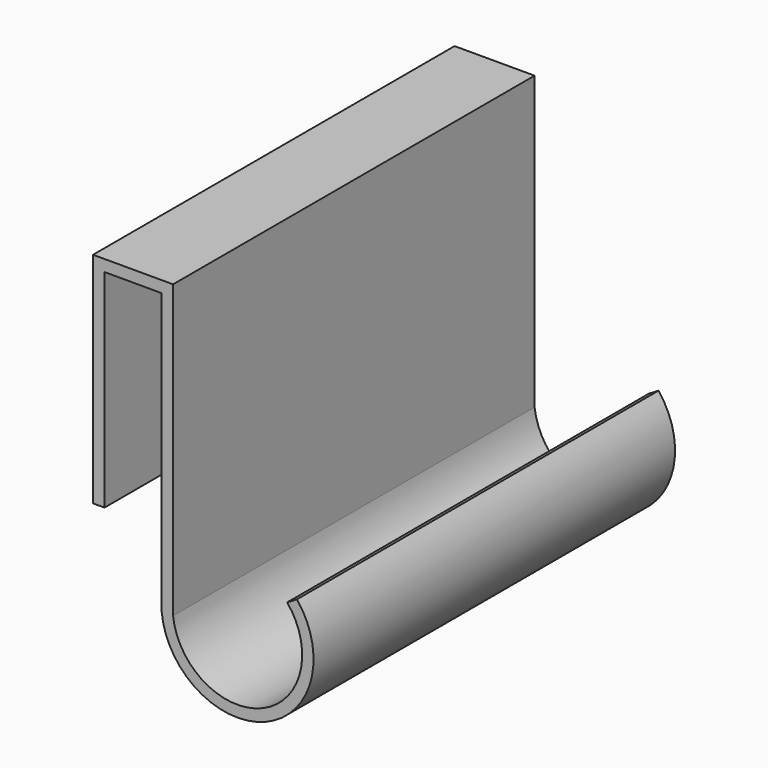
from build123d import *

# Parameters (mm, degrees)
F1_DEPTH = 99.56


# Not quite as in the source:
# - the program builds the solid bodies; features that only make, move or delete a surface that nothing else refers to are left out


with BuildPart() as f1:
    # F0 (on Front) → F1 (new body)
    with BuildSketch(Plane.XZ):
        with BuildLine():
            Line((-53.4761890293, -65.6504866451), (-40.9061890293, -65.6504866451))
            Line((-40.9061890293, -65.6504866451), (-40.9061890293, -127.2904866451))
            ThreePointArc((-40.9061890293, -127.2904866451), (-17.9599684542, -141.3452802415), (-11.0695237566, -115.3339743614))
            Line((-11.0695237566, -115.3339743614), (-13.2391586559, -116.635352248))
            ThreePointArc((-13.2391586559, -116.635352248), (-18.5765544792, -138.8900687432), (-38.3761890293, -127.4124961715))
            Line((-38.3761890293, -127.4124961715), (-38.3761890293, -63.1204866451))
            Line((-38.3761890293, -63.1204866451), (-56.0061890293, -63.1204866451))
            Line((-56.0061890293, -63.1204866451), (-56.0061890293, -111.3434480185))
            Line((-56.0061890293, -111.3434480185), (-53.4761890293, -111.3434480185))
            Line((-53.4761890293, -111.3434480185), (-53.4761890293, -65.6504866451))
        make_face()
    extrude(amount=F1_DEPTH)


solid = f1.part
